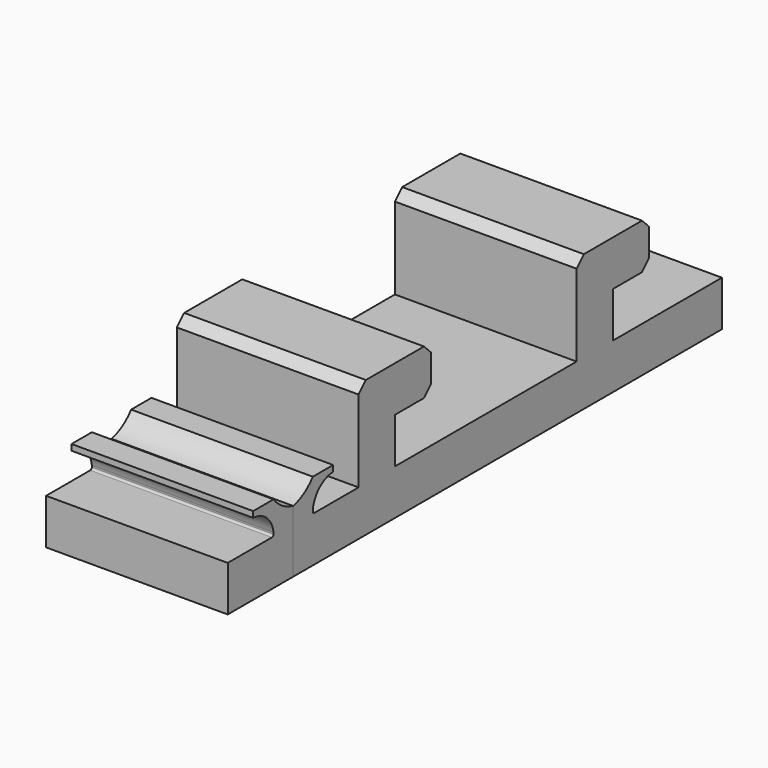
from build123d import *

# Parameters (mm, degrees)
F1_DEPTH = 20
F3_DEPTH = 20
F4_SIZE  = 1


# Not quite as in the source:
# - a pattern or mirror of a feature is missing from the dataset's text; its kind, count and spacing are read off the source's solid


with BuildPart() as f1:
    # F0 (on Right) → F1 (new body)
    with BuildSketch(Plane.YZ):
        with BuildLine():
            Line((5.5, 2.3115177173), (2.7, 2.3115177173))
            ThreePointArc((2.7, 2.3115177173), (1.5050999961, 1.2033549585), (0, 0.5784671916))
            Line((0, 0.5784671916), (0, -6.2862326842))
            Line((0, -6.2862326842), (9, -6.2862326842))
            Line((9, -6.2862326842), (9, -1.2862326842))
            Line((9, -1.2862326842), (2.9180552616, -1.2862326842))
            ThreePointArc((2.9180552616, -1.2862326842), (2.7638669074, -1.2223657768), (2.7, -1.0681774227))
            Line((2.7, -1.0681774227), (2.7, -0.9035626068))
            ThreePointArc((2.7, -0.9035626068), (3.6332473174, 0.8854712641), (5.5, 1.6515177173))
            Line((5.5, 1.6515177173), (5.5, 2.3115177173))
        make_face()
    extrude(amount=F1_DEPTH)


with BuildPart() as f1_copies_1:
    # F1_copies: instance of F1
    add(f1.part.mirror(Plane(origin=(0, 0, 0), x_dir=(0, 0, -1), z_dir=(0, -1, 0))))


with BuildPart() as f1_1:
    add(f1.part)

    # F2 (on Right) → F3 (join)
    with BuildSketch(Plane.YZ):
        Polygon((9, 8.7137673158), (9, -6.2862326842), (59, -6.2862326842), (59, -1.2862326842), (44, -1.2862326842), (44, 3.7137673158), (49, 3.7137673158), (49, 8.7137673158), (39, 8.7137673158), (39, -1.2862326842), (14, -1.2862326842), (14, 3.7137673158), (19, 3.7137673158), (19, 8.7137673158), align=None)
    extrude(amount=F3_DEPTH)

    # F4
    f4_edges = [f1_1.edges().sort_by_distance(p)[0] for p in [
        (10, 19, 3.713767),
        (10, 19, 8.713767),
        (10, 49, 8.713767),
        (10, 49, 3.713767),
        (10, 39, 8.713767),
        (10, 9, 8.713767),
    ]]
    chamfer(f4_edges, length=F4_SIZE)


solid = Compound([f1_copies_1.part, f1_1.part])
